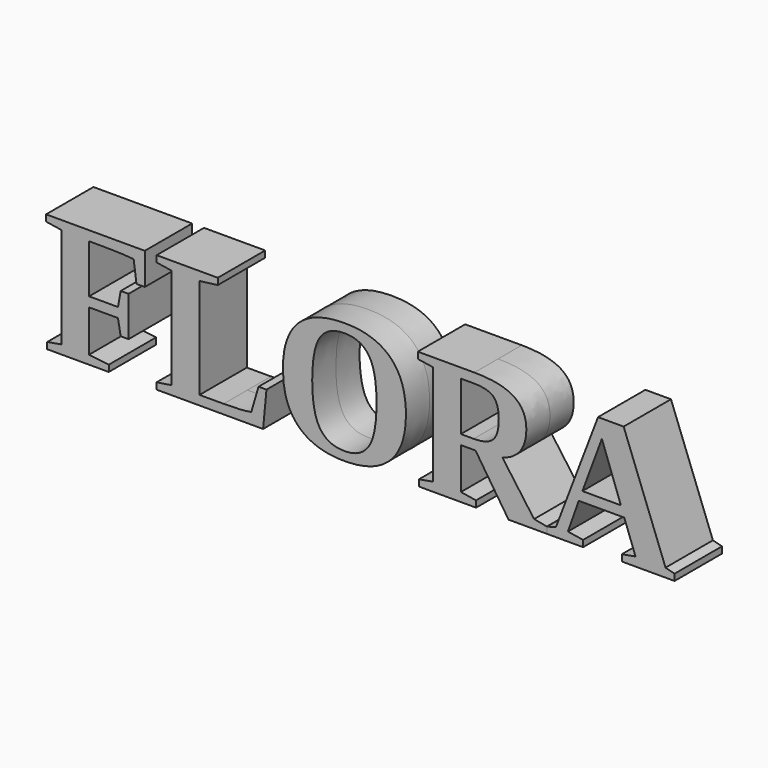
from build123d import *

# Parameters (mm, degrees)
F0_TEXT_SIZE = 77.588781197
F1_DEPTH     = 12.7


# Not quite as in the source:
# - Text() gives the source's letters only with a copy of the font that has no kerning and outlines rounded to 1/6400 em; it was checked with that copy


with BuildPart() as f1:
    # F0 (on Front) → F1 (new body, symmetric)
    with BuildSketch(Plane.XZ):
        with Locations((-176.2918904424, -21.2160758674)):
            Text('FLORA', F0_TEXT_SIZE, font='Tinos', font_style=FontStyle.BOLD, text_align=(TextAlign.LEFT, TextAlign.BOTTOM))
    extrude(amount=F1_DEPTH, both=True)


solid = f1.part
